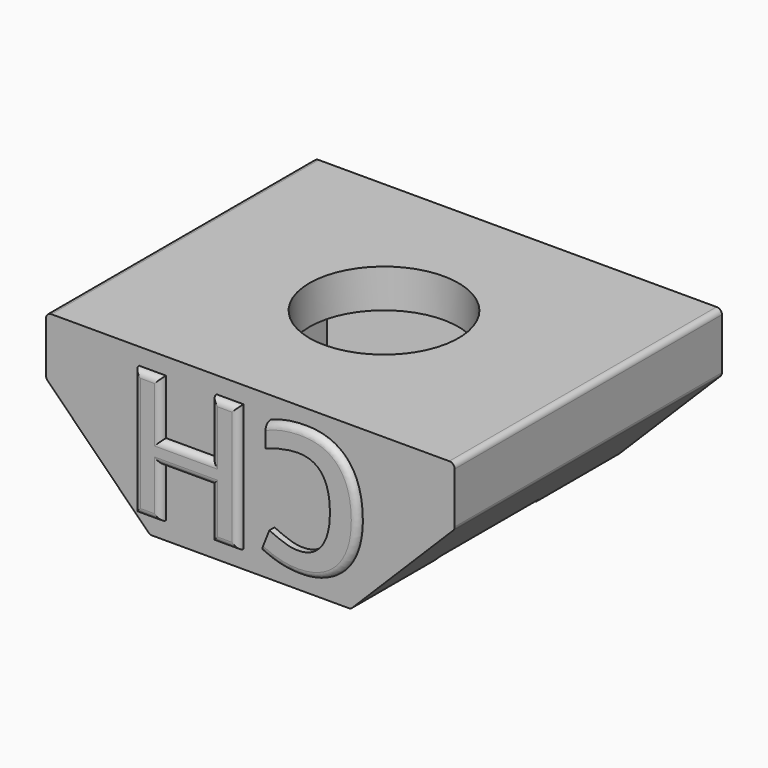
from build123d import *

# Parameters (mm, degrees)
F2_DEPTH     = 6.5
F5_DEPTH     = 4.808803
F6_D         = 5.8
F7_TEXT_SIZE = 6.9444444444
F8_DEPTH     = 0.25
F9_R         = 0.2499


# Not quite as in the source:
# - a fillet or chamfer is up to 0.001 mm smaller than in the source, because OpenCascade refuses the exact size
# - Text() gives the source's letters only with a copy of the font that has no kerning and outlines rounded to 1/6400 em; it was checked with that copy


with BuildPart() as f2:
    # F1 (on Front) → F2 (new body, symmetric)
    with BuildSketch(Plane.XZ):
        with BuildLine():
            Line((0, 12.442475), (-7.7389460073, 12.442475))
            ThreePointArc((-7.7389460073, 12.442475), (-7.8874364934, 12.3880458899), (-7.949967, 12.242781))
            Line((-7.949967, 12.242781), (-7.949967, 10.260188))
            ThreePointArc((-7.949967, 10.260188), (-7.9347430587, 10.1836520789), (-7.891388942, 10.118768058))
            Line((-7.8913889656, 10.1187680344), (-3.9658709656, 6.1932500344))
            ThreePointArc((-3.965870942, 6.193250058), (-3.9009869211, 6.1498959413), (-3.824451, 6.134672))
            Line((-3.824451, 6.134672), (0, 6.134672))
            Line((0, 6.134672), (3.824451, 6.134672))
            ThreePointArc((3.824451, 6.134672), (3.9009869211, 6.1498959413), (3.965870942, 6.193250058))
            Line((3.9658709656, 6.1932500344), (7.8913889656, 10.1187680344))
            ThreePointArc((7.891388942, 10.118768058), (7.9347430587, 10.1836520789), (7.949967, 10.260188))
            Line((7.949967, 10.260188), (7.949967, 12.242781))
            ThreePointArc((7.949967, 12.242781), (7.8874364934, 12.3880458899), (7.7389460073, 12.442475))
            Line((7.7389460073, 12.442475), (0, 12.442475))
        make_face()
    extrude(amount=F2_DEPTH, both=True)

    # F4 (on offset) → F5 (cut, through all)
    with BuildSketch(Plane.XY.offset(10.942475)):
        Polygon((4.125, 2.3815698604), (0, 4.7631397208), (-4.125, 2.3815698604), (-4.125, -2.3815698604), (0, -4.7631397208), (4.125, -2.3815698604), align=None)
    extrude(amount=-F5_DEPTH, mode=Mode.SUBTRACT)

    # F6 (through all)
    with Locations(Plane(origin=(0, 0, 10.942475), x_dir=(1, 0, 0), z_dir=(0, 0, -1))):
        with Locations((0, 0)):
            Hole(F6_D / 2)

    # F7 (on face) → F8 (join)
    with BuildSketch(Plane.XZ.offset(6.5)):
        with Locations(Location((4.7808159722, 11.7885735), (0, 0, 180))):
            Text('CH', F7_TEXT_SIZE, font='Open Sans', font_style=FontStyle.BOLD, text_align=(TextAlign.LEFT, TextAlign.BOTTOM))
    extrude(amount=F8_DEPTH)

    # F9 (radius 0.25 in the source; OpenCascade refuses exactly that, so slightly less here)
    f9_edges = [f2.edges().sort_by_distance(p)[0] for p in [
        (4.376352, -6.75, 9.233944),
        (-0.793728, -6.75, 6.830891),
        (-3.806424, -6.75, 6.830891),
        (-2.30089, -6.75, 8.774251),
        (-3.282335, -6.75, 7.802571),
        (-1.319444, -6.75, 7.802571),
        (-4.330512, -6.75, 9.309732),
        (-3.806424, -6.75, 11.788574),
        (-3.282335, -6.75, 10.718695),
        (-2.30089, -6.75, 9.648817),
        (-1.319444, -6.75, 10.718695),
        (-0.793728, -6.75, 11.788574),
        (-0.268012, -6.75, 9.309732),
    ]]
    fillet(f9_edges, radius=F9_R)


solid = f2.part
